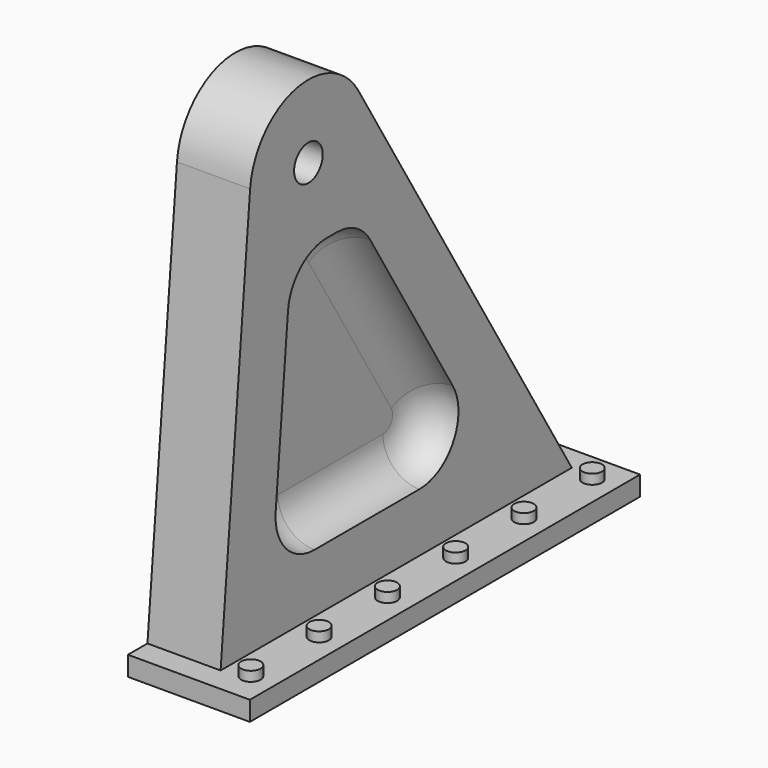
from build123d import *

# Parameters (mm, degrees)
F1_W      = 30
F1_H      = 1.2
F2_DEPTH  = 7.5
F3_R      = 1.1
F4_DEPTH  = 4.5
F6_DEPTH  = 2.25
F7_R      = 3
F8_R      = 2.24999
F9_R      = 0.6
F10_DEPTH = 0.6


# Not quite as in the source:
# - a fillet or chamfer is up to 0.001 mm smaller than in the source, because OpenCascade refuses the exact size


with BuildPart() as f2:
    # F1 (on Right) → F2 (new body)
    with BuildSketch(Plane.YZ):
        with Locations((6.75, 0.6)):
            Rectangle(F1_W, F1_H)
    extrude(amount=F2_DEPTH)

    # F3 (on Right) → F4 (join)
    with BuildSketch(Plane.YZ):
        with BuildLine():
            Line((-6.75, 1.2), (20.25, 1.2))
            Line((20.25, 1.2), (3.8491422789, 28.28111641))
            ThreePointArc((3.8491422789, 28.28111641), (-1.0140939829, 30.3342460462), (-4.4818163226, 26.3541317243))
            Line((-4.4818163226, 26.3541317243), (-6.75, 1.2))
        make_face()
        with Locations((0, 25.95)):
            Circle(F3_R, mode=Mode.SUBTRACT)
    extrude(amount=F4_DEPTH)

    # F5 (on face) → F6 (cut)
    with BuildSketch(Plane.YZ.offset(4.5)):
        Polygon((-1.3229485752, 21.3), (-2.8107769402, 4.8), (13.8610392149, 4.8), (3.8683140886, 21.3), align=None)
    extrude(amount=-F6_DEPTH, mode=Mode.SUBTRACT)

    # F7
    f7_edges = [f2.edges().sort_by_distance(p)[0] for p in [
        (3.375, -1.322949, 21.3),
        (3.375, 3.868314, 21.3),
        (3.375, 13.861039, 4.8),
        (3.375, -2.810777, 4.8),
    ]]
    fillet(f7_edges, radius=F7_R)

    # F8 (radius 2.25 in the source; OpenCascade refuses exactly that, so slightly less here)
    f8_edges = [f2.edges().sort_by_distance(p)[0] for p in [
        (2.25, 7.923497, 14.604078),
        (2.25, 11.150546, 6.327287),
        (2.25, 3.650611, 20.91364),
        (2.25, 4.504407, 4.8),
        (2.25, 1.798304, 21.3),
        (2.25, -1.742618, 5.776175),
        (2.25, -0.605116, 20.514527),
        (2.25, -2.042569, 13.319421),
    ]]
    fillet(f8_edges, radius=F8_R)

    # F9 (on face) → F10 (join)
    with BuildSketch(Plane.XY.offset(1.2)):
        with Locations((6, 19.95)):
            Circle(F9_R)
        with Locations((6, 14.7)):
            Circle(F9_R)
        with Locations((6, 9.45)):
            Circle(F9_R)
        with Locations((6, 4.2)):
            Circle(F9_R)
        with Locations((6, -1.05)):
            Circle(F9_R)
        with Locations((6, -6.3)):
            Circle(F9_R)
    extrude(amount=F10_DEPTH)


solid = f2.part
